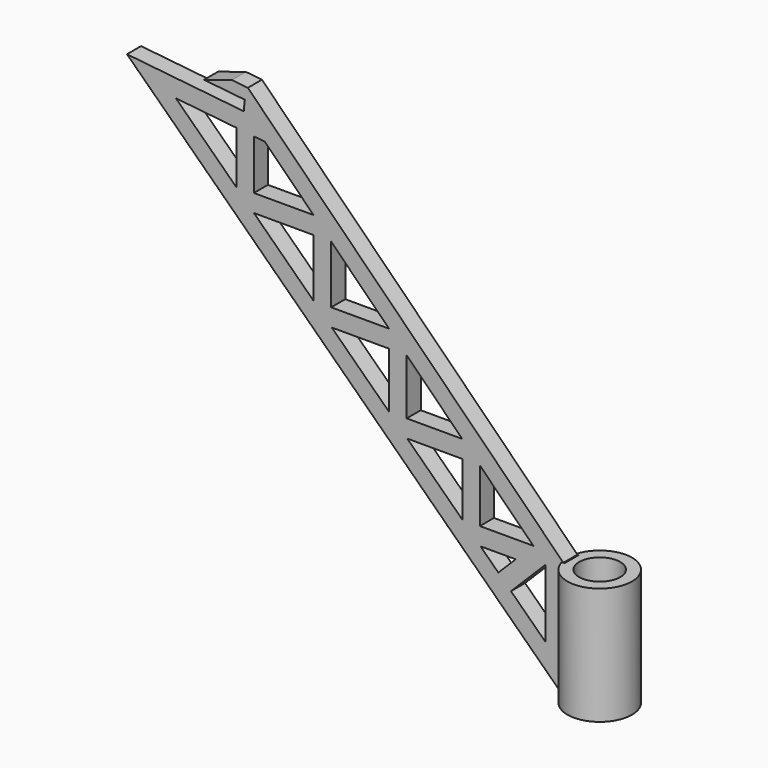
from build123d import *

# Parameters (mm, degrees)
F0_R     = 3.5
F1_DEPTH = 20
F3_DEPTH = 1.5


# Not quite as in the source:
# - a feature names something its author has since deleted; it is built from what else it names


with BuildPart() as f1:
    # F0 (on Top) → F1 (new body)
    with BuildSketch(Plane.XY):
        with BuildLine():
            Line((-4.7915026221, -1.5), (-5.2915026221, -1.5))
            ThreePointArc((-5.2915026221, -1.5), (5.5, 0), (-5.2915026221, 1.5))
            Line((-5.2915026221, 1.5), (-4.7915026221, 1.5))
            Line((-4.7915026221, 1.5), (-4.7915026221, -1.5))
        make_face()
        Circle(F0_R, mode=Mode.SUBTRACT)
    extrude(amount=F1_DEPTH)


with BuildPart() as f3:
    # F2 (on Front) → F3 (new body, symmetric)
    with BuildSketch(Plane.XZ):
        Polygon((-79.3605220673, 72.1106862647), (-5, 0), (-5, 20), (-54.4974746831, 69.4974746831), (-59.4700841599, 70.0201169994), align=None)
        Polygon((-57.7379381947, 66.8215362837), (-55.8675960947, 66.6249554076), (-47.5639026581, 58.321261971), (-44.5639026581, 55.321261971), (-34.6976905307, 45.4550498436), (-31.6976905307, 42.4550498436), (-22.2207557225, 32.9781150354), (-19.2207557225, 29.9781150354), (-10.1213203436, 20.8786796564), (-8, 18.7573593129), (-8, 7.0881840299), (-13.9242084231, 12.8331508898), (-16.0781127981, 14.9218872019), (-19.1271564551, 17.8786796564), (-22.2207557225, 20.8786796564), (-31.6040912633, 29.9781150354), (-34.6976905307, 32.9781150354), (-44.4703033907, 42.4550498436), (-47.5639026581, 45.4550498436), (-57.7379381947, 55.321261971), (-60.7379381947, 58.2304946227), (-71.0385888152, 68.2194909957), (-60.7379381947, 67.1368489895), align=None, mode=Mode.SUBTRACT)
        Polygon((-44.5639026581, 55.321261971), (-47.5639026581, 58.321261971), (-57.7379381947, 58.321261971), (-57.7379381947, 66.8215362837), (-60.7379381947, 67.1368489895), (-60.7379381947, 58.2304946227), (-57.7379381947, 55.321261971), (-47.5639026581, 55.321261971), (-47.5639026581, 45.4550498436), (-44.4703033907, 42.4550498436), (-34.6976905307, 42.4550498436), (-34.6976905307, 32.9781150354), (-31.6040912633, 29.9781150354), (-22.2207557225, 29.9781150354), (-22.2207557225, 20.8786796564), (-19.1271564551, 17.8786796564), (-13.1213203436, 17.8786796564), (-16.0781127981, 14.9218872019), (-13.9242084231, 12.8331508898), (-8, 18.7573593129), (-10.1213203436, 20.8786796564), (-19.2207557225, 20.8786796564), (-19.2207557225, 29.9781150354), (-22.2207557225, 32.9781150354), (-31.6976905307, 32.9781150354), (-31.6976905307, 42.4550498436), (-34.6976905307, 45.4550498436), (-44.5639026581, 45.4550498436), align=None)
        Polygon((-59.281932926, 71.8102564111), (-59.4700841599, 70.0201169994), (-54.4974746831, 69.4974746831), (-58.7671691133, 73.7671691133), (-61.4764084229, 74.0519216391), (-66.2435861936, 72.5419556539), align=None)
    extrude(amount=F3_DEPTH, both=True)


solid = Compound([f1.part, f3.part])
